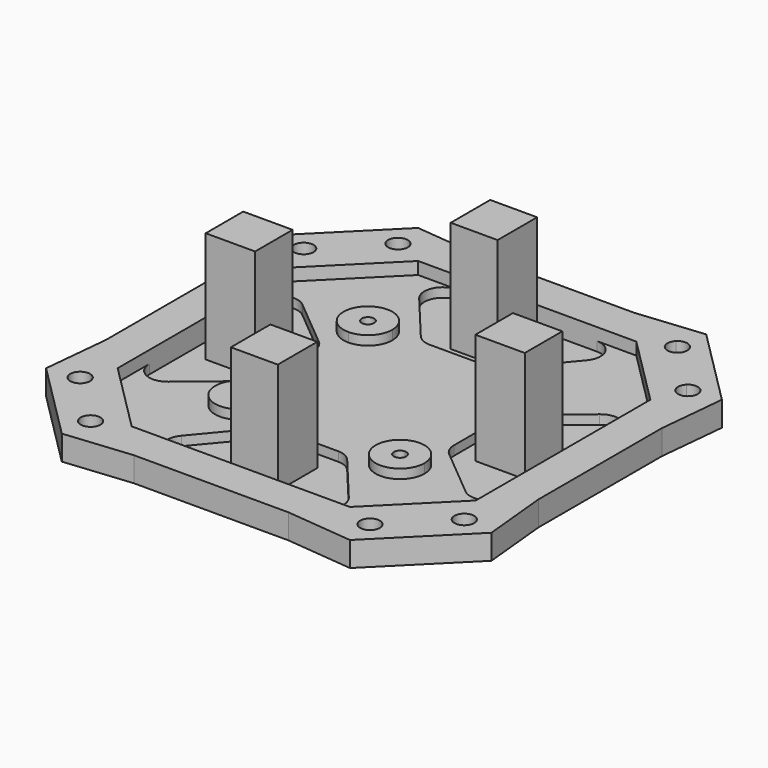
from build123d import *
from build123d import SkipClean  # not in build123d's __all__

# Parameters (mm, degrees)
F0_R      = 1.6
F1_DEPTH  = 4
F3_DEPTH  = 2
F5_DEPTH  = 1.5
F7_DEPTH  = 2.001
F8_DEPTH  = 25
F9_DEPTH  = 25
F10_DEPTH = 1.5
F11_W     = 8
F11_H     = 7.5978846649
F11_W_2   = 7.5978846649
F11_H_2   = 8
F12_DEPTH = 18


# Not quite as in the source:
# - after a boolean that leaves OpenCascade's solid faulty, fix() repairs it


with BuildPart() as f1:
    # F0 (on Top) → F1 (new body)
    with BuildSketch(Plane.XY):
        Polygon((0, 35), (0, 0), (26.8700576851, 26.8700576851), (29.6984848098, 29.6984848098), (23.3345237792, 36.0624458405), (12.5, 35), align=None)
        with BuildLine():
            ThreePointArc((24.227416998, 31.1126983722), (24.10562425, 30.5004048804), (23.7587878479, 29.9813275223))
            ThreePointArc((23.7587878479, 29.9813275223), (21.4960461481, 29.9813275223), (21.4960461481, 32.2440692221))
            ThreePointArc((21.4960461481, 32.2440692221), (23.2397104898, 32.5909056242), (24.227416998, 31.1126983722))
        make_face(mode=Mode.SUBTRACT)
        Polygon((0, -35), (0, 0), (0, 35), (-12.5, 35), (-23.3345237792, 36.0624458405), (-36.0624458405, 23.3345237792), (-35, 12.5), (-35, -12.5), (-36.0624458405, -23.3345237792), (-23.3345237792, -36.0624458405), (-12.5, -35), align=None)
        with Locations((-22.627416998, -31.1126983722)):
            Circle(F0_R, mode=Mode.SUBTRACT)
        with Locations((-31.1126983722, -22.627416998)):
            Circle(F0_R, mode=Mode.SUBTRACT)
        with Locations((-31.1126983722, 22.627416998)):
            Circle(F0_R, mode=Mode.SUBTRACT)
        with Locations((-22.627416998, 31.1126983722)):
            Circle(F0_R, mode=Mode.SUBTRACT)
        Polygon((26.8700576851, 26.8700576851), (0, 0), (0, -35), (12.5, -35), (23.3345237792, -36.0624458405), (36.0624458405, -23.3345237792), (35, -12.5), (35, 12.5), (36.0624458405, 23.3345237792), (29.6984848098, 29.6984848098), align=None)
        with Locations((22.627416998, -31.1126983722)):
            Circle(F0_R, mode=Mode.SUBTRACT)
        with Locations((31.1126983722, -22.627416998)):
            Circle(F0_R, mode=Mode.SUBTRACT)
        with BuildLine():
            ThreePointArc((32.2440692221, 21.4960461481), (29.9813275223, 21.4960461481), (29.9813275223, 23.7587878479))
            ThreePointArc((29.9813275223, 23.7587878479), (31.724991864, 24.10562425), (32.7126983722, 22.627416998))
            ThreePointArc((32.7126983722, 22.627416998), (32.5909056242, 22.0151235062), (32.2440692221, 21.4960461481))
        make_face(mode=Mode.SUBTRACT)
    extrude(amount=F1_DEPTH)

    # F2 (on face) → F3 (cut)
    with BuildSketch(Plane.XY.offset(4)):
        Polygon((-29, 17.6690475583), (-29, 0), (0, 0), (0, 29), (-17.6690475583, 29), align=None)
        Polygon((0, 0), (-29, 0), (-29, -17.6690475583), (-17.6690475583, -29), (17.6690475583, -29), (29, -17.6690475583), (29, 17.6690451666), (17.6690451666, 29), (0, 29), align=None)
    extrude(amount=-F3_DEPTH, mode=Mode.SUBTRACT)

    # F4 (on face) → F5 (cut)
    with BuildSketch(Plane.XY.offset(2)):
        with BuildLine():
            Line((-15, -4.5950587171), (-15, 0))
            Line((-15, 0), (-29, 0))
            Line((-29, 0), (-29, -11.2630858933))
            ThreePointArc((-29, -11.2630858933), (-27.2723298637, -13.979918004), (-24.0792155214, -13.5675569794))
            Line((-24.0792155214, -13.5675569794), (-16.0792155214, -6.8995298032))
            ThreePointArc((-16.0792155214, -6.8995298032), (-15.2831678893, -5.8673885808), (-15, -4.5950587171))
        make_face()
        with BuildLine():
            Line((-29, 0), (-15, 0))
            Line((-15, 0), (-15, 4.5950587171))
            ThreePointArc((-15, 4.5950587171), (-15.2831678893, 5.8673885808), (-16.0792155214, 6.8995298032))
            Line((-16.0792155214, 6.8995298032), (-24.0792155214, 13.5675569794))
            ThreePointArc((-24.0792155214, 13.5675569794), (-27.2723298637, 13.979918004), (-29, 11.2630858933))
            Line((-29, 11.2630858933), (-29, 0))
        make_face()
        with BuildLine():
            Line((0, 15), (0, 29))
            Line((0, 29), (-11.2630858933, 29))
            ThreePointArc((-11.2630858933, 29), (-13.979918004, 27.2723298637), (-13.5675569794, 24.0792155214))
            Line((-13.5675569794, 24.0792155214), (-6.8995298032, 16.0792155214))
            ThreePointArc((-6.8995298032, 16.0792155214), (-5.8673885808, 15.2831678893), (-4.5950587171, 15))
            Line((-4.5950587171, 15), (0, 15))
        make_face()
        with BuildLine():
            Line((11.2630858933, 29), (0, 29))
            Line((0, 29), (0, 15))
            Line((0, 15), (4.5950587171, 15))
            ThreePointArc((4.5950587171, 15), (5.8673885808, 15.2831678893), (6.8995298032, 16.0792155214))
            Line((6.8995298032, 16.0792155214), (13.5675569794, 24.0792155214))
            ThreePointArc((13.5675569794, 24.0792155214), (13.979918004, 27.2723298637), (11.2630858933, 29))
        make_face()
        with BuildLine():
            Line((15, 4.5950587171), (15, 0))
            Line((15, 0), (29, 0))
            Line((29, 0), (29, 11.2630858933))
            ThreePointArc((29, 11.2630858933), (27.2723298637, 13.979918004), (24.0792155214, 13.5675569794))
            Line((24.0792155214, 13.5675569794), (16.0792155214, 6.8995298032))
            ThreePointArc((16.0792155214, 6.8995298032), (15.2831678893, 5.8673885808), (15, 4.5950587171))
        make_face()
        with BuildLine():
            Line((29, 0), (15, 0))
            Line((15, 0), (15, -4.5950587171))
            ThreePointArc((15, -4.5950587171), (15.2831678893, -5.8673885808), (16.0792155214, -6.8995298032))
            Line((16.0792155214, -6.8995298032), (24.0792155214, -13.5675569794))
            ThreePointArc((24.0792155214, -13.5675569794), (27.2723298637, -13.979918004), (29, -11.2630858933))
            Line((29, -11.2630858933), (29, 0))
        make_face()
        with BuildLine():
            Line((4.5950587171, -15), (0, -15))
            Line((0, -15), (0, -29))
            Line((0, -29), (11.2630858933, -29))
            ThreePointArc((11.2630858933, -29), (13.979918004, -27.2723298637), (13.5675569794, -24.0792155214))
            Line((13.5675569794, -24.0792155214), (6.8995298032, -16.0792155214))
            ThreePointArc((6.8995298032, -16.0792155214), (5.8673885808, -15.2831678893), (4.5950587171, -15))
        make_face()
        with BuildLine():
            Line((0, -29), (0, -15))
            Line((0, -15), (-4.5950587171, -15))
            ThreePointArc((-4.5950587171, -15), (-5.8673885808, -15.2831678893), (-6.8995298032, -16.0792155214))
            Line((-6.8995298032, -16.0792155214), (-13.5675569794, -24.0792155214))
            ThreePointArc((-13.5675569794, -24.0792155214), (-13.979918004, -27.2723298637), (-11.2630858933, -29))
            Line((-11.2630858933, -29), (0, -29))
        make_face()
    extrude(amount=-F5_DEPTH, mode=Mode.SUBTRACT)

    # F6 (on face) → F7 (cut, through all)
    with BuildSketch(Plane.XY.offset(2)):
        with BuildLine():
            Line((13, 13), (13, 12))
            ThreePointArc((13, 12), (13.7071067812, 12.2928932188), (14, 13))
            ThreePointArc((14, 13), (13, 14), (12, 13))
            Line((12, 13), (13, 13))
        make_face()
        with BuildLine():
            ThreePointArc((12, 13), (12.2928932188, 12.2928932188), (13, 12))
            Line((13, 12), (13, 13))
            Line((13, 13), (12, 13))
        make_face()
    extrude(amount=-F7_DEPTH, mode=Mode.SUBTRACT)

    # F6 (on face) → F8 (cut)
    with BuildSketch(Plane.XY.offset(2)):
        with BuildLine():
            Line((0, 13), (0, 0))
            Line((0, 0), (13, 0))
            Line((13, 0), (13, 9.05))
            ThreePointArc((13, 9.05), (10.2069282143, 10.2069282143), (9.05, 13))
            Line((9.05, 13), (0, 13))
        make_face()
        with BuildLine():
            Line((-13, 0), (0, 0))
            Line((0, 0), (0, 13))
            Line((0, 13), (-9.05, 13))
            ThreePointArc((-9.05, 13), (-10.2069282143, 10.2069282143), (-13, 9.05))
            Line((-13, 9.05), (-13, 0))
        make_face()
        with BuildLine():
            Line((13, 0), (0, 0))
            Line((0, 0), (0, -13))
            Line((0, -13), (9.05, -13))
            ThreePointArc((9.05, -13), (10.2069282143, -10.2069282143), (13, -9.05))
            Line((13, -9.05), (13, 0))
        make_face()
        with BuildLine():
            Line((0, -13), (0, 0))
            Line((0, 0), (-13, 0))
            Line((-13, 0), (-13, -9.05))
            ThreePointArc((-13, -9.05), (-10.2069282143, -10.2069282143), (-9.05, -13))
            Line((-9.05, -13), (0, -13))
        make_face()
        with BuildLine():
            ThreePointArc((9.05, 13), (10.2069282143, 10.2069282143), (13, 9.05))
            Line((13, 9.05), (13, 12))
            ThreePointArc((13, 12), (12.2928932188, 12.2928932188), (12, 13))
            Line((12, 13), (9.05, 13))
        make_face()
        with BuildLine():
            Line((13, 12), (13, 9.05))
            ThreePointArc((13, 9.05), (15.7930717857, 10.2069282143), (16.95, 13))
            ThreePointArc((16.95, 13), (13, 16.95), (9.05, 13))
            Line((9.05, 13), (12, 13))
            ThreePointArc((12, 13), (13, 14), (14, 13))
            ThreePointArc((14, 13), (13.7071067812, 12.2928932188), (13, 12))
        make_face()
        with BuildLine():
            ThreePointArc((16.95, -13), (15.7930717857, -10.2069282143), (13, -9.05))
            Line((13, -9.05), (13, -12))
            ThreePointArc((13, -12), (13.7071067812, -12.2928932188), (14, -13))
            ThreePointArc((14, -13), (13, -14), (12, -13))
            Line((12, -13), (9.05, -13))
            ThreePointArc((9.05, -13), (13, -16.95), (16.95, -13))
        make_face()
        with BuildLine():
            Line((13, -12), (13, -9.05))
            ThreePointArc((13, -9.05), (10.2069282143, -10.2069282143), (9.05, -13))
            Line((9.05, -13), (12, -13))
            ThreePointArc((12, -13), (12.2928932188, -12.2928932188), (13, -12))
        make_face()
        with BuildLine():
            ThreePointArc((-13, 9.05), (-10.2069282143, 10.2069282143), (-9.05, 13))
            Line((-9.05, 13), (-12, 13))
            ThreePointArc((-12, 13), (-12.2928932188, 12.2928932188), (-13, 12))
            Line((-13, 12), (-13, 9.05))
        make_face()
        with BuildLine():
            Line((-12, 13), (-9.05, 13))
            ThreePointArc((-9.05, 13), (-15.7930717857, 15.7930717857), (-13, 9.05))
            Line((-13, 9.05), (-13, 12))
            ThreePointArc((-13, 12), (-13.7071067812, 13.7071067812), (-12, 13))
        make_face()
        with BuildLine():
            ThreePointArc((-13, -9.05), (-15.7930717857, -15.7930717857), (-9.05, -13))
            Line((-9.05, -13), (-12, -13))
            ThreePointArc((-12, -13), (-13.7071067812, -13.7071067812), (-13, -12))
            Line((-13, -12), (-13, -9.05))
        make_face()
        with BuildLine():
            Line((-12, -13), (-9.05, -13))
            ThreePointArc((-9.05, -13), (-10.2069282143, -10.2069282143), (-13, -9.05))
            Line((-13, -9.05), (-13, -12))
            ThreePointArc((-13, -12), (-12.2928932188, -12.2928932188), (-12, -13))
        make_face()
    extrude(amount=F8_DEPTH, mode=Mode.SUBTRACT)

    # F6 (on face) → F9 (cut)
    with BuildSketch(Plane.XY.offset(2)):
        with BuildLine():
            Line((-13, 13), (-12, 13))
            ThreePointArc((-12, 13), (-13.7071067812, 13.7071067812), (-13, 12))
            Line((-13, 12), (-13, 13))
        make_face()
        with BuildLine():
            ThreePointArc((-13, 12), (-12.2928932188, 12.2928932188), (-12, 13))
            Line((-12, 13), (-13, 13))
            Line((-13, 13), (-13, 12))
        make_face()
        with BuildLine():
            ThreePointArc((-13, -12), (-13.7071067812, -13.7071067812), (-12, -13))
            Line((-12, -13), (-13, -13))
            Line((-13, -13), (-13, -12))
        make_face()
        with BuildLine():
            Line((-13, -13), (-12, -13))
            ThreePointArc((-12, -13), (-12.2928932188, -12.2928932188), (-13, -12))
            Line((-13, -12), (-13, -13))
        make_face()
        with BuildLine():
            ThreePointArc((14, -13), (13.7071067812, -12.2928932188), (13, -12))
            Line((13, -12), (13, -13))
            Line((13, -13), (12, -13))
            ThreePointArc((12, -13), (13, -14), (14, -13))
        make_face()
        with BuildLine():
            Line((13, -13), (13, -12))
            ThreePointArc((13, -12), (12.2928932188, -12.2928932188), (12, -13))
            Line((12, -13), (13, -13))
        make_face()
        with BuildLine():
            ThreePointArc((12, 13), (12.2928932188, 12.2928932188), (13, 12))
            Line((13, 12), (13, 13))
            Line((13, 13), (12, 13))
        make_face()
        with BuildLine():
            Line((13, 13), (13, 12))
            ThreePointArc((13, 12), (13.7071067812, 12.2928932188), (14, 13))
            ThreePointArc((14, 13), (13, 14), (12, 13))
            Line((12, 13), (13, 13))
        make_face()
    extrude(amount=-F9_DEPTH, mode=Mode.SUBTRACT)

    # F6 (on face) → F10 (join)
    with BuildSketch(Plane.XY.offset(2)):
        with BuildLine():
            Line((-12, 13), (-9.05, 13))
            ThreePointArc((-9.05, 13), (-15.7930717857, 15.7930717857), (-13, 9.05))
            Line((-13, 9.05), (-13, 12))
            ThreePointArc((-13, 12), (-13.7071067812, 13.7071067812), (-12, 13))
        make_face()
        with BuildLine():
            ThreePointArc((-13, 9.05), (-10.2069282143, 10.2069282143), (-9.05, 13))
            Line((-9.05, 13), (-12, 13))
            ThreePointArc((-12, 13), (-12.2928932188, 12.2928932188), (-13, 12))
            Line((-13, 12), (-13, 9.05))
        make_face()
        with BuildLine():
            ThreePointArc((-13, -9.05), (-15.7930717857, -15.7930717857), (-9.05, -13))
            Line((-9.05, -13), (-12, -13))
            ThreePointArc((-12, -13), (-13.7071067812, -13.7071067812), (-13, -12))
            Line((-13, -12), (-13, -9.05))
        make_face()
        with BuildLine():
            Line((-12, -13), (-9.05, -13))
            ThreePointArc((-9.05, -13), (-10.2069282143, -10.2069282143), (-13, -9.05))
            Line((-13, -9.05), (-13, -12))
            ThreePointArc((-13, -12), (-12.2928932188, -12.2928932188), (-12, -13))
        make_face()
        with BuildLine():
            ThreePointArc((16.95, -13), (15.7930717857, -10.2069282143), (13, -9.05))
            Line((13, -9.05), (13, -12))
            ThreePointArc((13, -12), (13.7071067812, -12.2928932188), (14, -13))
            ThreePointArc((14, -13), (13, -14), (12, -13))
            Line((12, -13), (9.05, -13))
            ThreePointArc((9.05, -13), (13, -16.95), (16.95, -13))
        make_face()
        with BuildLine():
            Line((13, -12), (13, -9.05))
            ThreePointArc((13, -9.05), (10.2069282143, -10.2069282143), (9.05, -13))
            Line((9.05, -13), (12, -13))
            ThreePointArc((12, -13), (12.2928932188, -12.2928932188), (13, -12))
        make_face()
        with BuildLine():
            Line((13, 12), (13, 9.05))
            ThreePointArc((13, 9.05), (15.7930717857, 10.2069282143), (16.95, 13))
            ThreePointArc((16.95, 13), (13, 16.95), (9.05, 13))
            Line((9.05, 13), (12, 13))
            ThreePointArc((12, 13), (13, 14), (14, 13))
            ThreePointArc((14, 13), (13.7071067812, 12.2928932188), (13, 12))
        make_face()
        with BuildLine():
            ThreePointArc((9.05, 13), (10.2069282143, 10.2069282143), (13, 9.05))
            Line((13, 9.05), (13, 12))
            ThreePointArc((13, 12), (12.2928932188, 12.2928932188), (12, 13))
            Line((12, 13), (9.05, 13))
        make_face()
    with SkipClean():  # cleaning this boolean's faces spoils the solid; the shape is the same uncleaned
        extrude(amount=F10_DEPTH)

    # F11 (on face) → F12 (join)
    with BuildSketch(Plane.XY.offset(0.5)):
        with Locations((-22, 0.2010576676)):
            Rectangle(F11_W, F11_H)
        with Locations((-0.2010576676, -22)):
            Rectangle(F11_W_2, F11_H_2)
        with Locations((22, -0.2010576676)):
            Rectangle(F11_W, F11_H)
        with Locations((0.2010576676, 22)):
            Rectangle(F11_W_2, F11_H_2)
    extrude(amount=F12_DEPTH)

    add(f1.part.fix(), mode=Mode.REPLACE)


solid = f1.part
